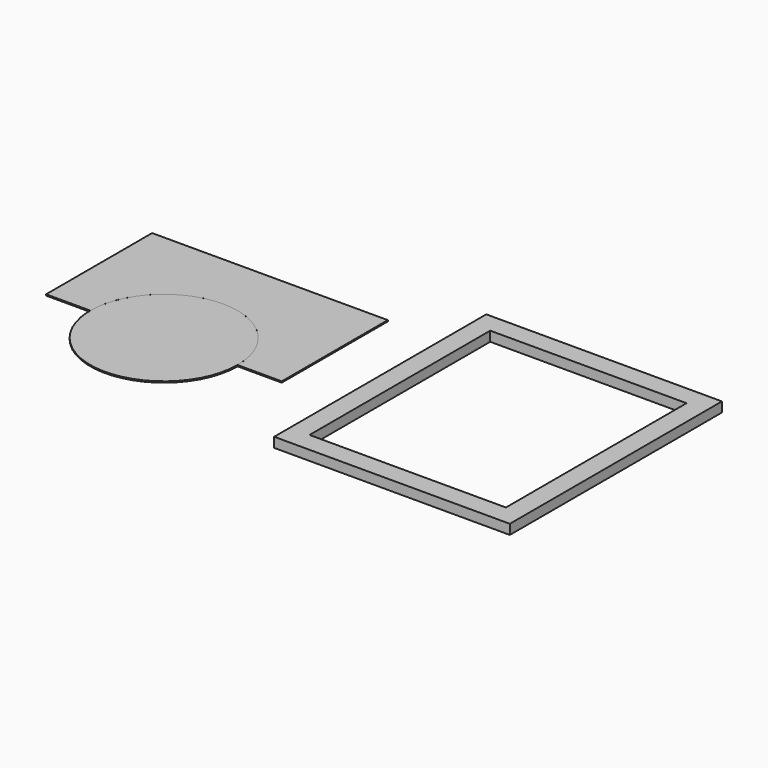
from build123d import *

# Parameters (mm, degrees)
F1_DEPTH = 3.175
F2_DEPTH = 3.175
F3_W     = 609.6
F3_H     = 685.8
F3_W_2   = 508
F3_H_2   = 584.2
F4_DEPTH = 25.4


# Not quite as in the source:
# - a length typed as a fraction of an inch, garbled in the dataset ("3 / 203.2 mm" for 3/8 in), is restored


with BuildPart() as f1:
    # F0 (on Top) → F1 (new body)
    with BuildSketch(Plane.XY):
        with BuildLine():
            ThreePointArc((-594.3986861706, 181.333437562), (-403.8986861706, -9.166562438), (-213.3986861706, 181.333437562))
            ThreePointArc((-213.3986861706, 181.333437562), (-403.8986861706, 371.833437562), (-594.3986861706, 181.333437562))
        make_face()
    extrude(amount=F1_DEPTH)


with BuildPart() as f2:
    # F0 (on Top) → F2 (new body)
    with BuildSketch(Plane.XY):
        with BuildLine():
            Line((-213.3986861706, 181.333437562), (-99.0986861706, 181.333437562))
            Line((-99.0986861706, 181.333437562), (-99.0986861706, 524.233437562))
            Line((-99.0986861706, 524.233437562), (-708.6986861706, 524.233437562))
            Line((-708.6986861706, 524.233437562), (-708.6986861706, 181.333437562))
            Line((-708.6986861706, 181.333437562), (-594.3986861706, 181.333437562))
            ThreePointArc((-594.3986861706, 181.333437562), (-403.8986861706, 371.833437562), (-213.3986861706, 181.333437562))
        make_face()
    extrude(amount=F2_DEPTH)


with BuildPart() as f4:
    # F3 (on Top) → F4 (new body)
    with BuildSketch(Plane.XY):
        with Locations((371.9603717327, 291.9999957085)):
            Rectangle(F3_W, F3_H)
        with Locations((371.9603717327, 291.9999957085)):
            Rectangle(F3_W_2, F3_H_2, mode=Mode.SUBTRACT)
    extrude(amount=F4_DEPTH)


solid = Compound([f1.part, f2.part, f4.part])
